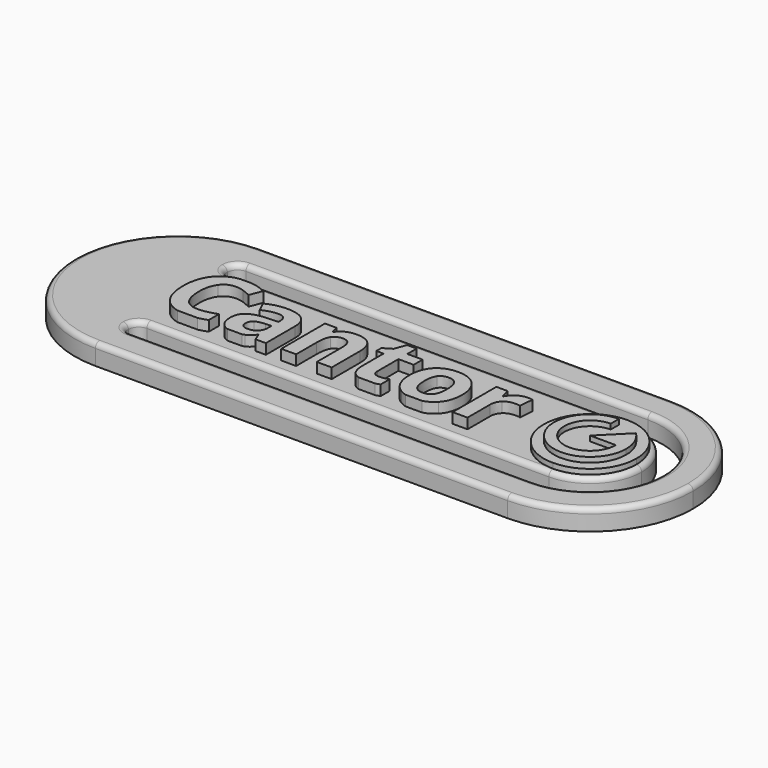
from build123d import *

# Parameters (mm, degrees)
F1_DEPTH = 2
F2_R     = 0.5
F4_DEPTH = 1
F6_DEPTH = 0.5
F8_DEPTH = 0.5


with BuildPart() as f1:
    # F0 (on Top) → F1 (new body)
    with BuildSketch(Plane.XY):
        with BuildLine():
            ThreePointArc((0, 10), (2.9289321881, 2.9289321881), (10, 0))
            Line((10, 0), (50, 0))
            ThreePointArc((50, 0), (57.0710678119, 2.9289321881), (60, 10))
            ThreePointArc((60, 10), (57.0710678119, 17.0710678119), (50, 20))
            Line((50, 20), (10, 20))
            ThreePointArc((10, 20), (2.9289321881, 17.0710678119), (0, 10))
        make_face()
        with BuildLine():
            Line((50, 3), (11, 3))
            ThreePointArc((11, 3), (10.2928932188, 3.2928932188), (10, 4))
            ThreePointArc((10, 4), (10.2928932188, 4.7071067812), (11, 5))
            Line((11, 5), (50, 5))
            ThreePointArc((50, 5), (53.5355339059, 6.4644660941), (55, 10))
            ThreePointArc((55, 10), (53.5355339059, 13.5355339059), (50, 15))
            Line((50, 15), (11, 15))
            ThreePointArc((11, 15), (10.2928932188, 15.2928932188), (10, 16))
            ThreePointArc((10, 16), (10.2928932188, 16.7071067812), (11, 17))
            Line((11, 17), (50, 17))
            ThreePointArc((50, 17), (54.9497474683, 14.9497474683), (57, 10))
            ThreePointArc((57, 10), (54.9497474683, 5.0502525317), (50, 3))
        make_face(mode=Mode.SUBTRACT)
    extrude(amount=F1_DEPTH)

    # F2
    f2_edges = [f1.edges().sort_by_distance(p)[0] for p in [
        (0, 10, 2),
        (30.5, 17, 2),
        (30, 0, 2),
        (60, 10, 2),
        (30, 20, 2),
        (30.5, 3, 2),
        (10, 4, 2),
        (30.5, 5, 2),
        (55, 10, 2),
        (30.5, 15, 2),
        (10, 16, 2),
        (57, 10, 2),
    ]]
    fillet(f2_edges, radius=F2_R)

    # F3 (on face) → F4 (join)
    with BuildSketch(Plane.XY.offset(2)):
        with BuildLine():
            Line((12.7805307431, 6.5), (14.7217743985, 6.5))
            add(Edge.make_bspline(
                [(15.591796875, 6.7612847222), (15.1801008351, 6.5891342429), (14.7217743985, 6.5)],
                knots=[0, 0, 0, 0.4822306436, 0.4822306436, 0.4822306436], degree=2))
            Line((15.591796875, 6.7612847222), (15.591796875, 7.9947916667))
            add(Edge.make_bspline(
                [(13.8220486111, 7.6302083333), (14.552734375, 7.6302083333), (15.591796875, 7.9947916667)],
                knots=[0, 0, 0, 1, 1, 1], degree=2))
            add(Edge.make_bspline(
                [(12.0796440972, 9.9513888889), (12.0796440972, 7.6302083333), (13.8220486111, 7.6302083333)],
                knots=[0, 0, 0, 1, 1, 1], degree=2))
            add(Edge.make_bspline(
                [(12.5353732639, 11.6907552083), (12.0796440972, 11.06640625), (12.0796440972, 9.9513888889)],
                knots=[0, 0, 0, 1, 1, 1], degree=2))
            add(Edge.make_bspline(
                [(13.8220486111, 12.3151041667), (12.9911024306, 12.3151041667), (12.5353732639, 11.6907552083)],
                knots=[0, 0, 0, 1, 1, 1], degree=2))
            add(Edge.make_bspline(
                [(14.5952690972, 12.1776258681), (14.2018229167, 12.3151041667), (13.8220486111, 12.3151041667)],
                knots=[0, 0, 0, 1, 1, 1], degree=2))
            add(Edge.make_bspline(
                [(15.3791232639, 11.8548177083), (14.9887152778, 12.0401475694), (14.5952690972, 12.1776258681)],
                knots=[0, 0, 0, 1, 1, 1], degree=2))
            Line((15.3791232639, 11.8548177083), (15.8530815972, 13.0518663194))
            add(Edge.make_bspline(
                [(14.3979145714, 13.5), (15.1227769369, 13.4007172063), (15.8530815972, 13.0518663194)],
                knots=[0.2845995164, 0.2845995164, 0.2845995164, 1, 1, 1], degree=2))
            Line((14.3979145714, 13.5), (13.2464473769, 13.5))
            add(Edge.make_bspline(
                [(12.091796875, 13.1057942708), (12.6072831166, 13.408615921), (13.2464473769, 13.5)],
                knots=[0, 0, 0, 0.6982247505, 0.6982247505, 0.6982247505], degree=2))
            add(Edge.make_bspline(
                [(10.9593098958, 11.8578559028), (11.353515625, 12.6720920139), (12.091796875, 13.1057942708)],
                knots=[0, 0, 0, 1, 1, 1], degree=2))
            add(Edge.make_bspline(
                [(10.5651041667, 9.9605034722), (10.5651041667, 11.0436197917), (10.9593098958, 11.8578559028)],
                knots=[0, 0, 0, 1, 1, 1], degree=2))
            add(Edge.make_bspline(
                [(11.3671875, 7.3233506944), (10.5651041667, 8.2424045139), (10.5651041667, 9.9605034722)],
                knots=[0, 0, 0, 1, 1, 1], degree=2))
            add(Edge.make_bspline(
                [(12.7805307431, 6.5), (11.9104423428, 6.700871187), (11.3671875, 7.3233506944)],
                knots=[0.3226952609, 0.3226952609, 0.3226952609, 1, 1, 1], degree=2))
        make_face()
        with BuildLine():
            Line((20.0442708333, 7.2215711806), (20.3253038194, 6.5))
            Line((20.3253038194, 6.5), (21.3355034722, 6.5))
            Line((21.3355034722, 6.5), (21.3355034722, 10.0364583333))
            add(Edge.make_bspline(
                [(20.7658420139, 11.4514973958), (21.3355034722, 10.9858940972), (21.3355034722, 10.0364583333)],
                knots=[0, 0, 0, 1, 1, 1], degree=2))
            add(Edge.make_bspline(
                [(19.1282552083, 11.9171006944), (20.1961805556, 11.9171006944), (20.7658420139, 11.4514973958)],
                knots=[0, 0, 0, 1, 1, 1], degree=2))
            add(Edge.make_bspline(
                [(17.0972222222, 11.4370659722), (18.0132378472, 11.9171006944), (19.1282552083, 11.9171006944)],
                knots=[0, 0, 0, 1, 1, 1], degree=2))
            Line((17.0972222222, 11.4370659722), (17.5757378472, 10.4587673611))
            add(Edge.make_bspline(
                [(19.0720486111, 10.8430989583), (18.435546875, 10.8430989583), (17.5757378472, 10.4587673611)],
                knots=[0, 0, 0, 1, 1, 1], degree=2))
            add(Edge.make_bspline(
                [(19.8984375, 10.0364583333), (19.8984375, 10.8430989583), (19.0720486111, 10.8430989583)],
                knots=[0, 0, 0, 1, 1, 1], degree=2))
            Line((19.8984375, 10.0364583333), (19.8984375, 9.8040364583))
            Line((19.8984375, 9.8040364583), (18.9763454861, 9.7751736111))
            add(Edge.make_bspline(
                [(17.1944444444, 9.3315972222), (17.7853732639, 9.7326388889), (18.9763454861, 9.7751736111)],
                knots=[0, 0, 0, 1, 1, 1], degree=2))
            add(Edge.make_bspline(
                [(16.603515625, 8.0859375), (16.603515625, 8.9305555556), (17.1944444444, 9.3315972222)],
                knots=[0, 0, 0, 1, 1, 1], degree=2))
            add(Edge.make_bspline(
                [(17.0425347222, 6.841796875), (16.603515625, 7.279296875), (16.603515625, 8.0859375)],
                knots=[0, 0, 0, 1, 1, 1], degree=2))
            add(Edge.make_bspline(
                [(17.6020168371, 6.5), (17.2762214384, 6.6089187633), (17.0425347222, 6.841796875)],
                knots=[0.4677071733, 0.4677071733, 0.4677071733, 1, 1, 1], degree=2))
            Line((17.6020168371, 6.5), (19.0301203125, 6.5))
            add(Edge.make_bspline(
                [(19.2543402778, 6.5827907986), (19.1506167656, 6.5349966312), (19.0301203125, 6.5)],
                knots=[0, 0, 0, 0.2677635541, 0.2677635541, 0.2677635541], degree=2))
            add(Edge.make_bspline(
                [(20.0062934028, 7.2215711806), (19.6417100694, 6.7612847222), (19.2543402778, 6.5827907986)],
                knots=[0, 0, 0, 1, 1, 1], degree=2))
            Line((20.0062934028, 7.2215711806), (20.0442708333, 7.2215711806))
        make_face()
        with BuildLine():
            Line((19.337890625, 8.9396701389), (19.8984375, 8.9594184028))
            Line((19.8984375, 8.9594184028), (19.8984375, 8.5219184028))
            add(Edge.make_bspline(
                [(19.5968967014, 7.7532552083), (19.8984375, 8.0434027778), (19.8984375, 8.5219184028)],
                knots=[0, 0, 0, 1, 1, 1], degree=2))
            add(Edge.make_bspline(
                [(18.791015625, 7.4631076389), (19.2953559028, 7.4631076389), (19.5968967014, 7.7532552083)],
                knots=[0, 0, 0, 1, 1, 1], degree=2))
            add(Edge.make_bspline(
                [(18.0891927083, 8.0768229167), (18.0891927083, 7.4631076389), (18.791015625, 7.4631076389)],
                knots=[0, 0, 0, 1, 1, 1], degree=2))
            add(Edge.make_bspline(
                [(18.3975694444, 8.7125651042), (18.0891927083, 8.5036892361), (18.0891927083, 8.0768229167)],
                knots=[0, 0, 0, 1, 1, 1], degree=2))
            add(Edge.make_bspline(
                [(19.337890625, 8.9396701389), (18.7059461806, 8.9214409722), (18.3975694444, 8.7125651042)],
                knots=[0, 0, 0, 1, 1, 1], degree=2))
        make_face(mode=Mode.SUBTRACT)
        with BuildLine():
            Line((22.8272569444, 11.8077256944), (22.8272569444, 6.5))
            Line((22.8272569444, 6.5), (24.2749565972, 6.5))
            Line((24.2749565972, 6.5), (24.2749565972, 8.9973958333))
            add(Edge.make_bspline(
                [(24.5453559028, 10.3433159722), (24.2749565972, 9.9377170139), (24.2749565972, 8.9973958333)],
                knots=[0, 0, 0, 1, 1, 1], degree=2))
            add(Edge.make_bspline(
                [(25.4233940972, 10.7489149306), (24.8157552083, 10.7489149306), (24.5453559028, 10.3433159722)],
                knots=[0, 0, 0, 1, 1, 1], degree=2))
            add(Edge.make_bspline(
                [(26.0743272569, 10.4618055556), (25.8700086806, 10.7489149306), (25.4233940972, 10.7489149306)],
                knots=[0, 0, 0, 1, 1, 1], degree=2))
            add(Edge.make_bspline(
                [(26.2786458333, 9.6004774306), (26.2786458333, 10.1746961806), (26.0743272569, 10.4618055556)],
                knots=[0, 0, 0, 1, 1, 1], degree=2))
            Line((26.2786458333, 9.6004774306), (26.2786458333, 6.5))
            Line((26.2786458333, 6.5), (27.7263454861, 6.5))
            Line((27.7263454861, 6.5), (27.7263454861, 9.9605034722))
            add(Edge.make_bspline(
                [(27.2470703125, 11.4059244792), (27.7263454861, 10.9053819444), (27.7263454861, 9.9605034722)],
                knots=[0, 0, 0, 1, 1, 1], degree=2))
            add(Edge.make_bspline(
                [(25.8411458333, 11.9064670139), (26.7677951389, 11.9064670139), (27.2470703125, 11.4059244792)],
                knots=[0, 0, 0, 1, 1, 1], degree=2))
            add(Edge.make_bspline(
                [(24.8757595486, 11.7097439236), (25.3003472222, 11.9064670139), (25.8411458333, 11.9064670139)],
                knots=[0, 0, 0, 1, 1, 1], degree=2))
            add(Edge.make_bspline(
                [(24.2081163194, 11.1286892361), (24.451171875, 11.5130208333), (24.8757595486, 11.7097439236)],
                knots=[0, 0, 0, 1, 1, 1], degree=2))
            Line((24.2081163194, 11.1286892361), (24.1276041667, 11.1286892361))
            Line((24.1276041667, 11.1286892361), (23.9331597222, 11.8077256944))
            Line((23.9331597222, 11.8077256944), (22.8272569444, 11.8077256944))
        make_face()
        with BuildLine():
            add(Edge.make_bspline(
                [(34.9073117771, 6.5), (34.5964263747, 6.5833410273), (34.3245442708, 6.7392578125)],
                knots=[0.5345224838, 0.5345224838, 0.5345224838, 1, 1, 1], degree=2))
            Line((34.9073117771, 6.5), (36.4850573236, 6.5))
            add(Edge.make_bspline(
                [(37.576171875, 7.1357421875), (37.1398474324, 6.6688750339), (36.4850573236, 6.5)],
                knots=[0, 0, 0, 0.6382803275, 0.6382803275, 0.6382803275], degree=2))
            add(Edge.make_bspline(
                [(38.259765625, 9.1629774306), (38.259765625, 7.8671875), (37.576171875, 7.1357421875)],
                knots=[0, 0, 0, 1, 1, 1], degree=2))
            add(Edge.make_bspline(
                [(37.9468315972, 10.6205512153), (38.259765625, 9.9984809028), (38.259765625, 9.1629774306)],
                knots=[0, 0, 0, 1, 1, 1], degree=2))
            add(Edge.make_bspline(
                [(37.0498046875, 11.5745442708), (37.6338975694, 11.2426215278), (37.9468315972, 10.6205512153)],
                knots=[0, 0, 0, 1, 1, 1], degree=2))
            add(Edge.make_bspline(
                [(35.7016059028, 11.9064670139), (36.4657118056, 11.9064670139), (37.0498046875, 11.5745442708)],
                knots=[0, 0, 0, 1, 1, 1], degree=2))
            add(Edge.make_bspline(
                [(33.7928602431, 11.1848958333), (34.4711371528, 11.9064670139), (35.7016059028, 11.9064670139)],
                knots=[0, 0, 0, 1, 1, 1], degree=2))
            add(Edge.make_bspline(
                [(33.1145833333, 9.1629774306), (33.1145833333, 10.4633246528), (33.7928602431, 11.1848958333)],
                knots=[0, 0, 0, 1, 1, 1], degree=2))
            add(Edge.make_bspline(
                [(33.4275173611, 7.7008463542), (33.1145833333, 8.3274739583), (33.1145833333, 9.1629774306)],
                knots=[0, 0, 0, 1, 1, 1], degree=2))
            add(Edge.make_bspline(
                [(34.3245442708, 6.7392578125), (33.7404513889, 7.07421875), (33.4275173611, 7.7008463542)],
                knots=[0, 0, 0, 1, 1, 1], degree=2))
        make_face()
        with BuildLine():
            add(Edge.make_bspline(
                [(34.5896267361, 9.1629774306), (34.5896267361, 8.3745659722), (34.8486328125, 7.9712456597)],
                knots=[0, 0, 0, 1, 1, 1], degree=2))
            add(Edge.make_bspline(
                [(34.8463541667, 10.3478732639), (34.5896267361, 9.9559461806), (34.5896267361, 9.1629774306)],
                knots=[0, 0, 0, 1, 1, 1], degree=2))
            add(Edge.make_bspline(
                [(35.6818576389, 10.7398003472), (35.1030815972, 10.7398003472), (34.8463541667, 10.3478732639)],
                knots=[0, 0, 0, 1, 1, 1], degree=2))
            add(Edge.make_bspline(
                [(36.5226779514, 10.3455946181), (36.2667100694, 10.7398003472), (35.6818576389, 10.7398003472)],
                knots=[0, 0, 0, 1, 1, 1], degree=2))
            add(Edge.make_bspline(
                [(36.7786458333, 9.1629774306), (36.7786458333, 9.9513888889), (36.5226779514, 10.3455946181)],
                knots=[0, 0, 0, 1, 1, 1], degree=2))
            add(Edge.make_bspline(
                [(36.5249565972, 7.9689670139), (36.7786458333, 8.3700086806), (36.7786458333, 9.1629774306)],
                knots=[0, 0, 0, 1, 1, 1], degree=2))
            add(Edge.make_bspline(
                [(35.6909722222, 7.5679253472), (36.2712673611, 7.5679253472), (36.5249565972, 7.9689670139)],
                knots=[0, 0, 0, 1, 1, 1], degree=2))
            add(Edge.make_bspline(
                [(34.8486328125, 7.9712456597), (35.1076388889, 7.5679253472), (35.6909722222, 7.5679253472)],
                knots=[0, 0, 0, 1, 1, 1], degree=2))
        make_face(mode=Mode.SUBTRACT)
        with BuildLine():
            add(Edge.make_bspline(
                [(30.3270546786, 6.5), (29.9810580734, 6.6094509408), (29.76953125, 6.8440755208)],
                knots=[0.4664939231, 0.4664939231, 0.4664939231, 1, 1, 1], degree=2))
            Line((30.3270546786, 6.5), (31.926890205, 6.5))
            add(Edge.make_bspline(
                [(32.3641493056, 6.6473524306), (32.1626991297, 6.5568130257), (31.926890205, 6.5)],
                knots=[0, 0, 0, 0.3725049801, 0.3725049801, 0.3725049801], degree=2))
            Line((32.3641493056, 6.6473524306), (32.3641493056, 7.7243923611))
            add(Edge.make_bspline(
                [(31.4526909722, 7.5588107639), (31.8324652778, 7.5588107639), (32.3641493056, 7.7243923611)],
                knots=[0, 0, 0, 1, 1, 1], degree=2))
            add(Edge.make_bspline(
                [(30.9939236111, 7.7061631944), (31.1671006944, 7.5588107639), (31.4526909722, 7.5588107639)],
                knots=[0, 0, 0, 1, 1, 1], degree=2))
            add(Edge.make_bspline(
                [(30.8207465278, 8.1618923611), (30.8207465278, 7.853515625), (30.9939236111, 7.7061631944)],
                knots=[0, 0, 0, 1, 1, 1], degree=2))
            Line((30.8207465278, 8.1618923611), (30.8207465278, 10.7200520833))
            Line((30.8207465278, 10.7200520833), (32.3064236111, 10.7200520833))
            Line((32.3064236111, 10.7200520833), (32.3064236111, 11.8077256944))
            Line((32.3064236111, 11.8077256944), (30.8207465278, 11.8077256944))
            Line((30.8207465278, 11.8077256944), (30.8207465278, 12.9379340278))
            Line((30.8207465278, 12.9379340278), (29.8956163194, 12.9379340278))
            Line((29.8956163194, 12.9379340278), (29.4778645833, 11.8168402778))
            Line((29.4778645833, 11.8168402778), (28.6803385417, 11.3322482639))
            Line((28.6803385417, 11.3322482639), (28.6803385417, 10.7200520833))
            Line((28.6803385417, 10.7200520833), (29.373046875, 10.7200520833))
            Line((29.373046875, 10.7200520833), (29.373046875, 8.1618923611))
            add(Edge.make_bspline(
                [(29.76953125, 6.8440755208), (29.373046875, 7.2838541667), (29.373046875, 8.1618923611)],
                knots=[0, 0, 0, 1, 1, 1], degree=2))
        make_face()
        with BuildLine():
            Line((39.4568142361, 11.8077256944), (39.4568142361, 6.5))
            Line((39.4568142361, 6.5), (40.9045138889, 6.5))
            Line((40.9045138889, 6.5), (40.9045138889, 9.2009548611))
            add(Edge.make_bspline(
                [(41.2918836806, 10.1982421875), (40.9045138889, 9.8420138889), (40.9045138889, 9.2009548611)],
                knots=[0, 0, 0, 1, 1, 1], degree=2))
            add(Edge.make_bspline(
                [(42.3719618056, 10.5544704861), (41.6792534722, 10.5544704861), (41.2918836806, 10.1982421875)],
                knots=[0, 0, 0, 1, 1, 1], degree=2))
            add(Edge.make_bspline(
                [(42.798828125, 10.5073784722), (42.6226128472, 10.5544704861), (42.3719618056, 10.5544704861)],
                knots=[0, 0, 0, 1, 1, 1], degree=2))
            Line((42.798828125, 10.5073784722), (42.908203125, 11.8639322917))
            add(Edge.make_bspline(
                [(42.4190538194, 11.9064670139), (42.7137586806, 11.9064670139), (42.908203125, 11.8639322917)],
                knots=[0, 0, 0, 1, 1, 1], degree=2))
            add(Edge.make_bspline(
                [(41.5053168403, 11.6337890625), (41.9253472222, 11.9064670139), (42.4190538194, 11.9064670139)],
                knots=[0, 0, 0, 1, 1, 1], degree=2))
            add(Edge.make_bspline(
                [(40.8376736111, 10.9144965278), (41.0852864583, 11.3611111111), (41.5053168403, 11.6337890625)],
                knots=[0, 0, 0, 1, 1, 1], degree=2))
            Line((40.8376736111, 10.9144965278), (40.7677951389, 10.9144965278))
            Line((40.7677951389, 10.9144965278), (40.5536024306, 11.8077256944))
            Line((40.5536024306, 11.8077256944), (39.4568142361, 11.8077256944))
        make_face()
    extrude(amount=F4_DEPTH)

    # F5 (on face) → F6 (join)
    with BuildSketch(Plane.XY.offset(2)):
        with BuildLine():
            ThreePointArc((50, 5.5), (53.1819805153, 6.8180194847), (54.5, 10))
            ThreePointArc((54.5, 10), (53.1819805153, 13.1819805153), (50, 14.5))
            ThreePointArc((50, 14.5), (45.5, 10), (50, 5.5))
        make_face()
    extrude(amount=F6_DEPTH)

    # F7 (on face) → F8 (join)
    with BuildSketch(Plane.XY.offset(2.5)):
        with BuildLine():
            ThreePointArc((50, 13.5), (47.5251262658, 7.5251262658), (53.5, 10))
            Line((53.5, 10), (52.5, 10))
            ThreePointArc((52.5, 10), (48.232233047, 8.232233047), (50, 12.5))
            Line((50, 12.5), (50, 13.5))
        make_face()
        with BuildLine():
            Line((50, 10), (52.5, 10))
            ThreePointArc((52.5, 10), (52.3096988313, 10.9567085809), (51.767766953, 11.767766953))
            Line((51.767766953, 11.767766953), (50, 10))
        make_face()
        with BuildLine():
            Line((52.5, 10), (53.5, 10))
            ThreePointArc((53.5, 10), (53.2335783638, 11.3393920133), (52.4748737342, 12.4748737342))
            Line((52.4748737342, 12.4748737342), (51.767766953, 11.767766953))
            ThreePointArc((51.767766953, 11.767766953), (52.3096988313, 10.9567085809), (52.5, 10))
        make_face()
    extrude(amount=F8_DEPTH)


solid = f1.part
